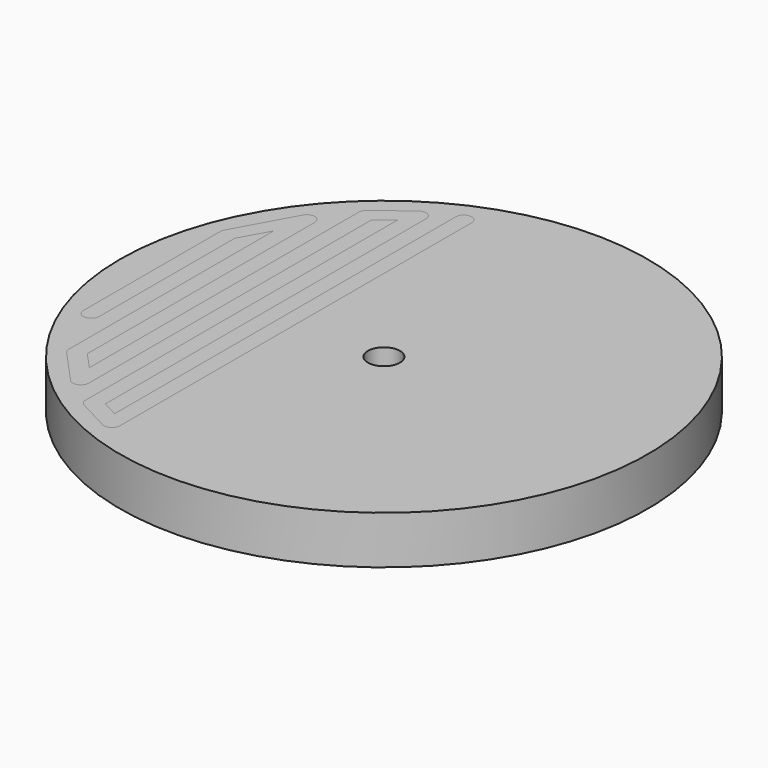
from build123d import *

# Parameters (mm, degrees)
F1_ANGLE = 30
F2_ANGLE = 30
F6_W     = 5
F6_H     = 200
F6_W_2   = 10
F8_DEPTH = 15


# Not quite as in the source:
# - a feature of the source that left no trace in its solid (it failed there, or was rolled back) is left out


with BuildPart() as f1:
    # F0 (on Front) → F1 (revolve)
    with BuildSketch(Plane.XZ):
        with BuildLine():
            Line((-147.1, 6.5387912874), (-152.8044866935, 6.5387912874))
            Line((-152.8044866935, 6.5387912874), (-157.8541755513, 6.5387912874))
            Line((-157.8541755513, 6.5387912874), (-159.5578471827, 6.5387912874))
            Line((-159.5578471827, 6.5387912874), (-164.874945747, 6.5387912874))
            Line((-164.874945747, 6.5387912874), (-164.874945747, 1.4487328955))
            Line((-164.874945747, 1.4487328955), (-164.874945747, -23.4612087126))
            Line((-164.874945747, -23.4612087126), (-10, -23.4612087126))
            Line((-10, -23.4612087126), (-10, -7.7473968267))
            Line((-10, -7.7473968267), (-10, -3.4612087126))
            Line((-10, -3.4612087126), (-10, 1.5387912874))
            Line((-10, 1.5387912874), (-17.5, 1.5387912874))
            Line((-17.5, 1.5387912874), (-19.8618033989, 6.2623980851))
            ThreePointArc((-19.8618033989, 6.2623980851), (-20.0461514383, 6.4641166916), (-20.3090169944, 6.5387912874))
            Line((-20.3090169944, 6.5387912874), (-30, 6.5387912874))
            Line((-30, 6.5387912874), (-147.1, 6.5387912874))
        make_face()
        with BuildLine():
            Line((-157.8541755513, 6.5387912874), (-152.8044866935, 6.5387912874))
            ThreePointArc((-152.8044866935, 6.5387912874), (-152.9974801055, 6.6091098931), (-153.1, 6.7871010014))
            Line((-153.1, 6.7871010014), (-153.3424612123, 8.173251478))
            ThreePointArc((-153.3424612123, 8.173251478), (-153.4108078086, 8.2919122169), (-153.5394700833, 8.3387912874))
            Line((-153.5394700833, 8.3387912874), (-154.3905712497, 8.3387912874))
            Line((-154.3905712497, 8.3387912874), (-155.2416724161, 8.3387912874))
            ThreePointArc((-155.2416724161, 8.3387912874), (-155.3650870202, 8.3192762877), (-155.4764594446, 8.2626354647))
            Line((-155.4764594446, 8.2626354647), (-157.8541755513, 6.5387912874))
        make_face()
    revolve(axis=Axis((0, 0, -0.2536289394), (0, 0, -1)), revolution_arc=F1_ANGLE)


with BuildPart() as f2:
    # F0 (on Front) → F2 (revolve)
    with BuildSketch(Plane.XZ):
        with BuildLine():
            ThreePointArc((-153.1, 6.7871010014), (-152.9974801055, 6.6091098931), (-152.8044866935, 6.5387912874))
            Line((-152.8044866935, 6.5387912874), (-147.1, 6.5387912874))
            Line((-147.1, 6.5387912874), (-30, 6.5387912874))
            Line((-30, 6.5387912874), (-20.3090169944, 6.5387912874))
            ThreePointArc((-20.3090169944, 6.5387912874), (-20.0461514383, 6.4641166916), (-19.8618033989, 6.2623980851))
            Line((-19.8618033989, 6.2623980851), (-17.5, 1.5387912874))
            Line((-17.5, 1.5387912874), (-10, 1.5387912874))
            Line((-10, 1.5387912874), (-10, 4.5176767256))
            Line((-10, 4.5176767256), (-17.2533747416, 4.5176767256))
            ThreePointArc((-17.2533747416, 4.5176767256), (-17.7791058537, 4.6670259172), (-18.1478019326, 5.0704631301))
            Line((-18.1478019326, 5.0704631301), (-18.9673762079, 6.7096116806))
            ThreePointArc((-18.9673762079, 6.7096116806), (-19.5204203262, 7.3147674999), (-20.3090169944, 7.5387912874))
            Line((-20.3090169944, 7.5387912874), (-30, 7.5387912874))
            Line((-30, 7.5387912874), (-147.1, 7.5387912874))
            Line((-147.1, 7.5387912874), (-152.2163006593, 7.5387912874))
            Line((-152.2163006593, 7.5387912874), (-152.4442840123, 8.8421718593))
            ThreePointArc((-152.4442840123, 8.8421718593), (-152.6493238012, 9.198154076), (-153.0353106254, 9.3387912874))
            Line((-153.0353106254, 9.3387912874), (-155.2416724161, 9.3387912874))
            ThreePointArc((-155.2416724161, 9.3387912874), (-155.6736235307, 9.2704887885), (-156.0634270161, 9.0722459081))
            Line((-156.0634270161, 9.0722459081), (-159.5578471827, 6.5387912874))
            Line((-159.5578471827, 6.5387912874), (-157.8541755513, 6.5387912874))
            Line((-157.8541755513, 6.5387912874), (-155.4764594446, 8.2626354647))
            ThreePointArc((-155.4764594446, 8.2626354647), (-155.3650870202, 8.3192762877), (-155.2416724161, 8.3387912874))
            Line((-155.2416724161, 8.3387912874), (-154.3905712497, 8.3387912874))
            Line((-154.3905712497, 8.3387912874), (-153.5394700833, 8.3387912874))
            ThreePointArc((-153.5394700833, 8.3387912874), (-153.4108078086, 8.2919122169), (-153.3424612123, 8.173251478))
            Line((-153.3424612123, 8.173251478), (-153.1, 6.7871010014))
        make_face()
    revolve(axis=Axis((0, 0, -0.2536289394), (0, 0, -1)), revolution_arc=F2_ANGLE)


with BuildPart() as f2_1:
    # F3: moved
    add(f2.part)


with BuildPart() as f4:
    # F0 (on Front) → F4 (revolve)
    with BuildSketch(Plane.XZ):
        with BuildLine():
            Line((-164.874945747, 6.5387912874), (-159.5578471827, 6.5387912874))
            Line((-159.5578471827, 6.5387912874), (-156.0634270161, 9.0722459081))
            ThreePointArc((-156.0634270161, 9.0722459081), (-155.6736235307, 9.2704887885), (-155.2416724161, 9.3387912874))
            Line((-155.2416724161, 9.3387912874), (-153.0353106254, 9.3387912874))
            ThreePointArc((-153.0353106254, 9.3387912874), (-152.6493238012, 9.198154076), (-152.4442840123, 8.8421718593))
            Line((-152.4442840123, 8.8421718593), (-152.2163006593, 7.5387912874))
            Line((-152.2163006593, 7.5387912874), (-147.1, 7.5387912874))
            Line((-147.1, 7.5387912874), (-147.1, 9.3387912874))
            Line((-147.1, 9.3387912874), (-30, 9.3387912874))
            Line((-30, 9.3387912874), (-30, 7.5387912874))
            Line((-30, 7.5387912874), (-20.3090169944, 7.5387912874))
            ThreePointArc((-20.3090169944, 7.5387912874), (-19.5204203262, 7.3147674999), (-18.9673762079, 6.7096116806))
            Line((-18.9673762079, 6.7096116806), (-18.1478019326, 5.0704631301))
            ThreePointArc((-18.1478019326, 5.0704631301), (-17.7791058537, 4.6670259172), (-17.2533747416, 4.5176767256))
            Line((-17.2533747416, 4.5176767256), (-10, 4.5176767256))
            Line((-10, 4.5176767256), (-10, 8.3387912874))
            Line((-10, 8.3387912874), (-10, 36.5387912874))
            Line((-10, 36.5387912874), (-164.874945747, 36.5387912874))
            Line((-164.874945747, 36.5387912874), (-164.874945747, 6.5387912874))
        make_face()
    revolve(axis=Axis((0, 0, -0.2536289394), (0, 0, -1)))


with BuildPart() as f4_1:
    # F5: moved
    add(f4.part)


with BuildPart() as f8:
    # F6 (on face) → F8 (new body)
    with BuildSketch(Plane.XY.offset(36.5387912874)):
        with BuildLine():
            Line((-85, 100), (-75, 100))
            Line((-75, 100), (-75, 126.737916042))
            ThreePointArc((-75, 126.737916042), (-77.9262502449, 131.2875931683), (-83.2798247813, 130.5118727725))
            Line((-83.2798247813, 130.5118727725), (-103.0111488123, 115.6271790176))
            ThreePointArc((-103.0111488123, 115.6271790176), (-104.4752510578, 113.8653918465), (-105, 111.6355649543))
            Line((-105, 111.6355649543), (-105, -98.7669287982))
            Line((-105, -98.7669287982), (-115, -87.8478189262))
            Line((-115, -87.8478189262), (-115, 89.7914214314))
            ThreePointArc((-115, 89.7914214314), (-118.7540322851, 94.6336899548), (-124.3790257813, 92.2047455303))
            Line((-124.3790257813, 92.2047455303), (-144.3399912833, 55.9851666545))
            ThreePointArc((-144.3399912833, 55.9851666545), (-144.8321815165, 54.7868621817), (-145, 53.5023304414))
            Line((-145, 53.5023304414), (-145, -53.5023304414))
            ThreePointArc((-145, -53.5023304414), (-140, -58.5023304414), (-135, -53.5023304414))
            Line((-135, -53.5023304414), (-135, 52.2144599446))
            Line((-135, 52.2144599446), (-125, 70.3596638287))
            Line((-125, 70.3596638287), (-125, -89.7914214314))
            ThreePointArc((-125, -89.7914214314), (-124.6602883929, -91.6029710704), (-123.6873151621, -93.1683589338))
            Line((-123.6873151621, -93.1683589338), (-103.819429446, -114.8623216397))
            ThreePointArc((-103.819429446, -114.8623216397), (-98.2820284097, -116.3311558239), (-95, -111.6355649543))
            Line((-95, -111.6355649543), (-95, -100))
            Line((-95, -100), (-100, -100))
            Line((-100, -100), (-100, 100))
            Line((-100, 100), (-95, 100))
            Line((-95, 100), (-95, 109.144278026))
            Line((-95, 109.144278026), (-85, 116.6879652776))
            Line((-85, 116.6879652776), (-85, 100))
        make_face()
        with Locations((-97.5, 0)):
            Rectangle(F6_W, F6_H)
        with Locations((-80, 0)):
            Rectangle(F6_W_2, F6_H)
        with BuildLine():
            Line((-55, -137.3408146279), (-55, -100))
            Line((-55, -100), (-65, -100))
            Line((-65, -100), (-65, -129.0130452242))
            Line((-65, -129.0130452242), (-75, -123.7257049977))
            Line((-75, -123.7257049977), (-75, -100))
            Line((-75, -100), (-85, -100))
            Line((-85, -100), (-85, -126.737916042))
            ThreePointArc((-85, -126.737916042), (-84.2828432022, -129.3180815609), (-82.337098358, -131.1580937833))
            Line((-82.337098358, -131.1580937833), (-62.7664257697, -141.5057742269))
            ThreePointArc((-62.7664257697, -141.5057742269), (-57.6369647536, -141.7471809795), (-55, -137.3408146279))
        make_face()
        with Locations((-60, 0)):
            Rectangle(F6_W_2, F6_H)
        with BuildLine():
            Line((-65, 100), (-55, 100))
            Line((-55, 100), (-55, 137.3408146279))
            ThreePointArc((-55, 137.3408146279), (-60, 142.3408146279), (-65, 137.3408146279))
            Line((-65, 137.3408146279), (-65, 100))
        make_face()
    extrude(amount=-F8_DEPTH)


solid = Compound([f1.part, f2_1.part, f4_1.part, f8.part])
